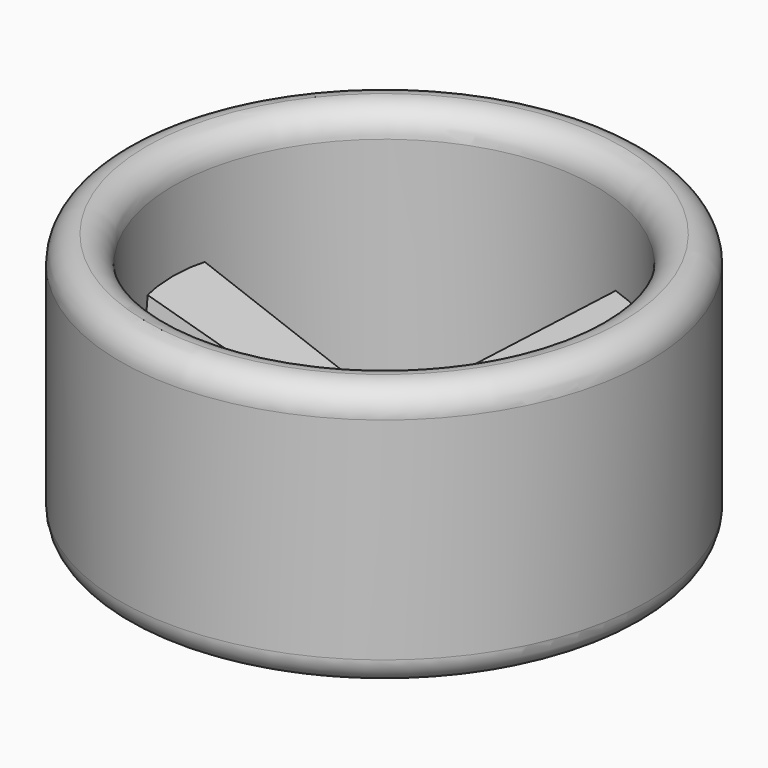
from build123d import *

# Parameters (mm, degrees)
F2_R      = 50
F2_R_2    = 40
F3_DEPTH  = 50
F0_R      = 5.0478433235
F4_DEPTH  = 4
F5_DEPTH  = 7
F0_R_2    = 2
F6_DEPTH  = 58.6
F7_R      = 4.99999
F8_R      = 4.99999
F9_DEPTH  = 4
F10_SIZE2 = 6.99999
F10_SIZE  = 1.875634
F11_DEPTH = 36.4222936332
F11_TAPER = -3
F12_DEPTH = 35.6510207057
F12_TAPER = -3
F13_DEPTH = 36.2196154892
F13_TAPER = -3


# Not quite as in the source:
# - a fillet or chamfer is up to 0.001 mm smaller than in the source, because OpenCascade refuses the exact size


with BuildPart() as f3:
    # F2 (on offset) → F3 (new body)
    with BuildSketch(Plane.XY.offset(30)):
        Circle(F2_R)
        Circle(F2_R_2, mode=Mode.SUBTRACT)
    extrude(amount=-F3_DEPTH)

    # F0 (on Top) → F6 (cut)
    with BuildSketch(Plane.XY):
        Circle(F0_R_2)
    extrude(amount=F6_DEPTH, mode=Mode.SUBTRACT)

    # F7 (radius 5 in the source; OpenCascade refuses exactly that, so slightly less here)
    f7_edges = [f3.edges().sort_by_distance(p)[0] for p in [
        (-40, 0, -20),
        (-50, 0, -20),
    ]]
    fillet(f7_edges, radius=F7_R)

    # F8 (radius 5 in the source; OpenCascade refuses exactly that, so slightly less here)
    f8_edges = [f3.edges().sort_by_distance(p)[0] for p in [
        (-40, 0, 30),
        (-50, 0, 30),
    ]]
    fillet(f8_edges, radius=F8_R)


with BuildPart() as f4:
    # F0 (on Top) → F4 (new body)
    with BuildSketch(Plane.XY):
        Polygon((6.135, -3.5420439015), (6.135, 3.5420439015), (0, 7.084087803), (-6.135, 3.5420439015), (-6.135, -3.5420439015), (0, -7.084087803), align=None)
        Circle(F0_R, mode=Mode.SUBTRACT)
    extrude(amount=-F4_DEPTH)

    # F0 (on Top) → F5 (join)
    with BuildSketch(Plane.XY):
        Polygon((11.135, -6.4287952474), (11.135, 6.4287952474), (0, 12.8575904949), (-11.135, 6.4287952474), (-11.135, -6.4287952474), (0, -12.8575904949), align=None)
        Polygon((0, 7.084087803), (6.135, 3.5420439015), (6.135, -3.5420439015), (0, -7.084087803), (-6.135, -3.5420439015), (-6.135, 3.5420439015), align=None, mode=Mode.SUBTRACT)
    extrude(amount=-F5_DEPTH)

    # F0 (on Top) → F9 (join)
    with BuildSketch(Plane.XY):
        Circle(F0_R)
        Circle(F0_R_2, mode=Mode.SUBTRACT)
    extrude(amount=-F9_DEPTH)

    # F10 (size 1.875644347 and 7 in the source; OpenCascade refuses exactly that, so slightly less here)
    f10_edges = [f4.edges().sort_by_distance(p)[0] for p in [
        (-5.5675, -9.643193, 0),
        (5.5675, 9.643193, 0),
        (11.135, 0, 0),
        (-11.135, 0, 0),
        (-5.5675, 9.643193, 0),
        (5.5675, -9.643193, 0),
    ]]
    f10_side = f4.faces().sort_by_distance((5.39741, -9.348588, 0))[0]
    chamfer(f10_edges, length=F10_SIZE, length2=F10_SIZE2, reference=f10_side)


with BuildPart() as f11:
    # F10_face (on face) → F11 (new body)
    with BuildSketch(Plane(origin=(5.1129663969, 8.8559175768, -3.6072911298), x_dir=(-0.8660254038, 0.5, 0), z_dir=(0.4829630454, 0.8365165328, 0.2588180579))):
        Polygon((-5.3458974526, 3.7345415598), (-6.4287952474, -3.5123793658), (6.4287952474, -3.5123793658), (5.3458974526, 3.7345415598), align=None)
    extrude(amount=F11_DEPTH, taper=F11_TAPER)


with BuildPart() as f12:
    # F10_face1 (on face) → F12 (new body)
    with BuildSketch(Plane(origin=(5.1129663969, -8.8559175768, -3.6072911298), x_dir=(0.8660254038, 0.5, 0), z_dir=(0.4829630454, -0.8365165328, 0.2588180579))):
        Polygon((-5.3458974526, 3.7345415598), (-6.4287952474, -3.5123793658), (6.4287952474, -3.5123793658), (5.3458974526, 3.7345415598), align=None)
    extrude(amount=F12_DEPTH, taper=F12_TAPER)


with BuildPart() as f13:
    # F10_face2 (on face) → F13 (new body)
    with BuildSketch(Plane(origin=(-10.2259327938, 0, -3.6072911298), x_dir=(0, -1, 0), z_dir=(-0.9659260908, 0, 0.2588180579))):
        Polygon((-5.3458974526, 3.7345415598), (-6.4287952474, -3.5123793658), (6.4287952474, -3.5123793658), (5.3458974526, 3.7345415598), align=None)
    extrude(amount=F13_DEPTH, taper=F13_TAPER)


solid = Compound([f3.part, f4.part, f11.part, f12.part, f13.part])
